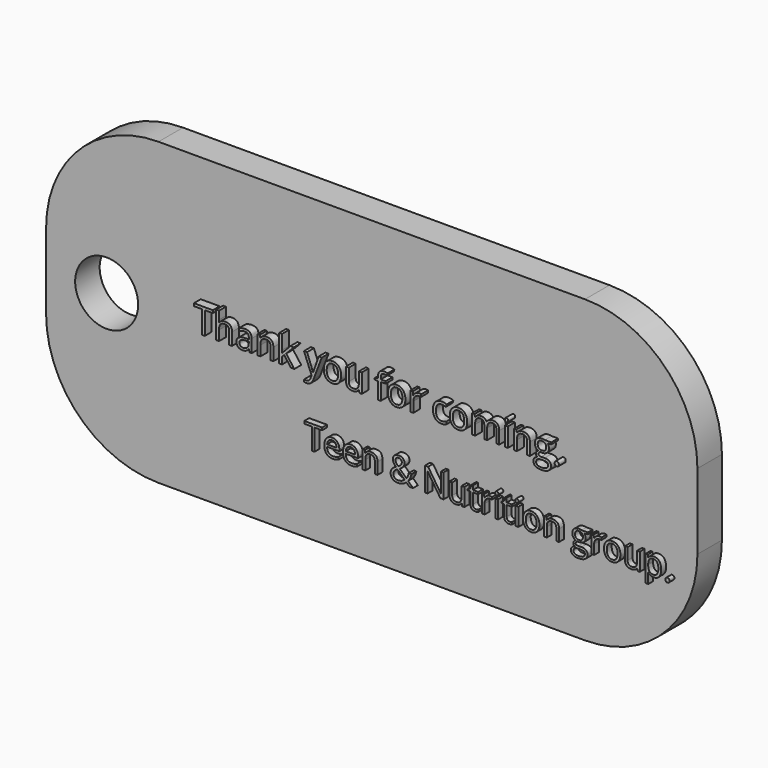
from build123d import *

# Parameters (mm, degrees)
F0_W         = 135.0143402815
F0_H         = 62.2506998479
F1_DEPTH     = 3.175
F2_R         = 23.301989304
F3_R         = 6.5242055925
F4_DEPTH     = 12.7
F5_TEXT_SIZE = 7.3298964424
F6_DEPTH     = 1.778
F7_TEXT_SIZE = 6.8972930162
F8_DEPTH     = 1.27


# Not quite as in the source:
# - Text() gives the source's letters only with a copy of the font that has no kerning and outlines rounded to 1/6400 em; it was checked with that copy


with BuildPart() as f1:
    # F0 (on Front) → F1 (new body, symmetric)
    with BuildSketch(Plane.XZ):
        Rectangle(F0_W, F0_H)
    extrude(amount=F1_DEPTH, both=True)

    # F2
    f2_edges = [f1.edges().sort_by_distance(p)[0] for p in [
        (-67.50717, 0, 31.12535),
        (67.50717, 0, -31.12535),
        (67.50717, 0, 31.12535),
        (-67.50717, 0, -31.12535),
    ]]
    fillet(f2_edges, radius=F2_R)

    # F3 (on Front) → F4 (cut, symmetric)
    with BuildSketch(Plane.XZ):
        with Locations((-54.9515224993, 0)):
            Circle(F3_R)
    extrude(amount=F4_DEPTH, both=True, mode=Mode.SUBTRACT)

    # F5 (on face) → F6 (join)
    with BuildSketch(Plane.XZ.offset(3.175)):
        with Locations((-35.5141610845, 0)):
            Text('Thank you for coming.', F5_TEXT_SIZE, font='Open Sans', text_align=(TextAlign.LEFT, TextAlign.BOTTOM))
    extrude(amount=F6_DEPTH)

    # F7 (on face) → F8 (join)
    with BuildSketch(Plane.XZ.offset(3.175)):
        with Locations((-13.0317651826, -14.0786297195)):
            Text('Teen & Nutrition group.', F7_TEXT_SIZE, font='Open Sans', text_align=(TextAlign.LEFT, TextAlign.BOTTOM))
    extrude(amount=F8_DEPTH)


solid = f1.part
